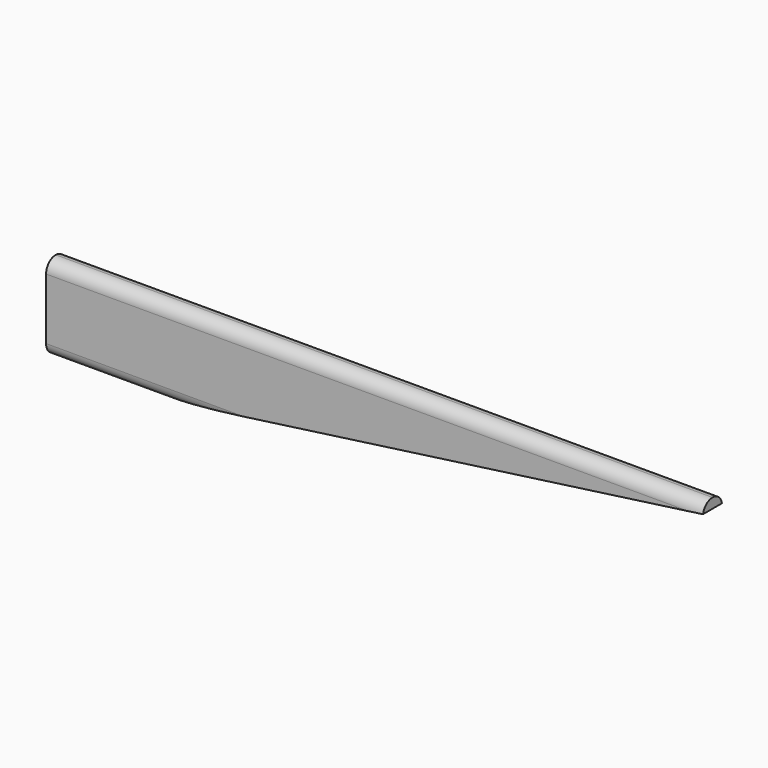
from build123d import *

# Parameters (mm, degrees)
F1_DEPTH = 3.5
F2_R     = 3.49999


# Not quite as in the source:
# - a fillet or chamfer is up to 0.001 mm smaller than in the source, because OpenCascade refuses the exact size


with BuildPart() as f1:
    # F0 (on Front) → F1 (new body, symmetric)
    with BuildSketch(Plane.XZ):
        Polygon((192, 0), (0, 0), (0, -24.9), (32.5, -24.9), (192, -2.9), align=None)
    extrude(amount=F1_DEPTH, both=True)

    # F2 (radius 3.5 in the source; OpenCascade refuses exactly that, so slightly less here)
    f2_edges = [f1.edges().sort_by_distance(p)[0] for p in [
        (96, -3.5, 0),
        (96, 3.5, 0),
        (16.25, -3.5, -24.9),
        (16.25, 3.5, -24.9),
    ]]
    fillet(f2_edges, radius=F2_R)


solid = f1.part
